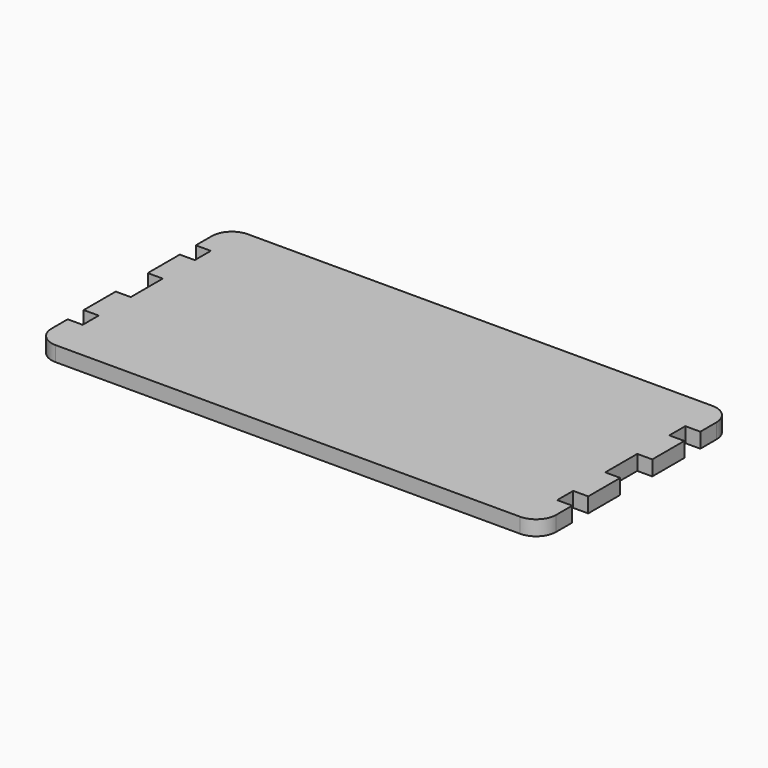
from build123d import *

# Parameters (mm, degrees)
F1_DEPTH = 4.7625


# Not quite as in the source:
# - a length typed as a fraction of an inch, garbled in the dataset ("3 / 203.2 mm" for 3/8 in), is restored
# - a feature names something its author has since deleted; it is built from what else it names


with BuildPart() as f1:
    # F0 (on Top) → F1 (new body)
    with BuildSketch(Plane.XY):
        with BuildLine():
            ThreePointArc((0, 6.35), (1.8598719395, 1.8598719395), (6.35, 0))
            Line((6.35, 0), (80.01, 0))
            Line((80.01, 0), (153.67, 0))
            ThreePointArc((153.67, 0), (158.1601280605, 1.8598719395), (160.02, 6.35))
            Line((160.02, 6.35), (160.02, 12.7))
            Line((160.02, 12.7), (155.2575, 12.7))
            Line((155.2575, 12.7), (155.2575, 19.05))
            Line((155.2575, 19.05), (160.02, 19.05))
            Line((160.02, 19.05), (160.02, 31.75))
            Line((160.02, 31.75), (155.2575, 31.75))
            Line((155.2575, 31.75), (155.2575, 44.45))
            Line((155.2575, 44.45), (160.02, 44.45))
            Line((160.02, 44.45), (160.02, 57.15))
            Line((160.02, 57.15), (155.2575, 57.15))
            Line((155.2575, 57.15), (155.2575, 63.5))
            Line((155.2575, 63.5), (160.02, 63.5))
            Line((160.02, 63.5), (160.02, 69.85))
            ThreePointArc((160.02, 69.85), (158.1601280605, 74.3401280605), (153.67, 76.2))
            Line((153.67, 76.2), (80.01, 76.2))
            Line((80.01, 76.2), (6.35, 76.2))
            ThreePointArc((6.35, 76.2), (1.8598719395, 74.3401280605), (0, 69.85))
            Line((0, 69.85), (0, 63.5))
            Line((0, 63.5), (4.7625, 63.5))
            Line((4.7625, 63.5), (4.7625, 57.15))
            Line((4.7625, 57.15), (0, 57.15))
            Line((0, 57.15), (0, 44.45))
            Line((0, 44.45), (4.7625, 44.45))
            Line((4.7625, 44.45), (4.7625, 31.75))
            Line((4.7625, 31.75), (0, 31.75))
            Line((0, 31.75), (0, 19.05))
            Line((0, 19.05), (4.7625, 19.05))
            Line((4.7625, 19.05), (4.7625, 12.7))
            Line((4.7625, 12.7), (0, 12.7))
            Line((0, 12.7), (0, 6.35))
        make_face()
    extrude(amount=F1_DEPTH)


solid = f1.part
